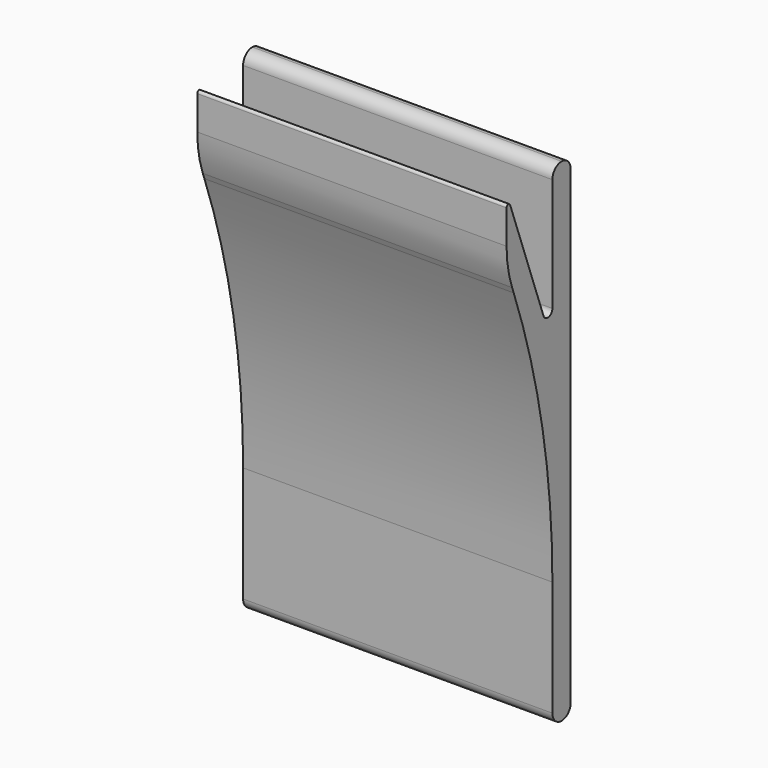
from build123d import *

# Parameters (mm, degrees)
F0_W     = 27
F0_H     = 43
F1_DEPTH = 2
F3_DEPTH = 27
F4_R     = 70
F5_R     = 0.5
F6_R     = 10
F7_R     = 0.99999
F8_R     = 0.2


# Not quite as in the source:
# - a fillet or chamfer is up to 0.001 mm smaller than in the source, because OpenCascade refuses the exact size


with BuildPart() as f1:
    # F0 (on Front) → F1 (new body)
    with BuildSketch(Plane.XZ):
        with Locations((13.5, 21.5)):
            Rectangle(F0_W, F0_H)
    extrude(amount=F1_DEPTH)

    # F2 (on Right) → F3 (join, through all)
    with BuildSketch(Plane.YZ):
        Polygon((0, 17.9200492635), (0, 23.7676580638), (-7, 43), (-7, 37.1523911997), align=None)
    extrude(amount=F3_DEPTH)

    # F4
    f4_edges = [f1.edges().sort_by_distance(p)[0] for p in [
        (13.5, -2, 23.415004),
    ]]
    fillet(f4_edges, radius=F4_R)

    # F5
    f5_edges = [f1.edges().sort_by_distance(p)[0] for p in [
        (13.5, -2, 29.262613),
    ]]
    fillet(f5_edges, radius=F5_R)

    # F6
    f6_edges = [f1.edges().sort_by_distance(p)[0] for p in [
        (13.5, -7, 37.152391),
    ]]
    fillet(f6_edges, radius=F6_R)

    # F7 (radius 1 in the source; OpenCascade refuses exactly that, so slightly less here)
    f7_edges = [f1.edges().sort_by_distance(p)[0] for p in [
        (13.5, -2, 43),
        (13.5, 0, 43),
        (13.5, -2, 0),
        (13.5, 0, 0),
    ]]
    fillet(f7_edges, radius=F7_R)

    # F8
    f8_edges = [f1.edges().sort_by_distance(p)[0] for p in [
        (13.5, -7, 43),
    ]]
    fillet(f8_edges, radius=F8_R)


solid = f1.part
